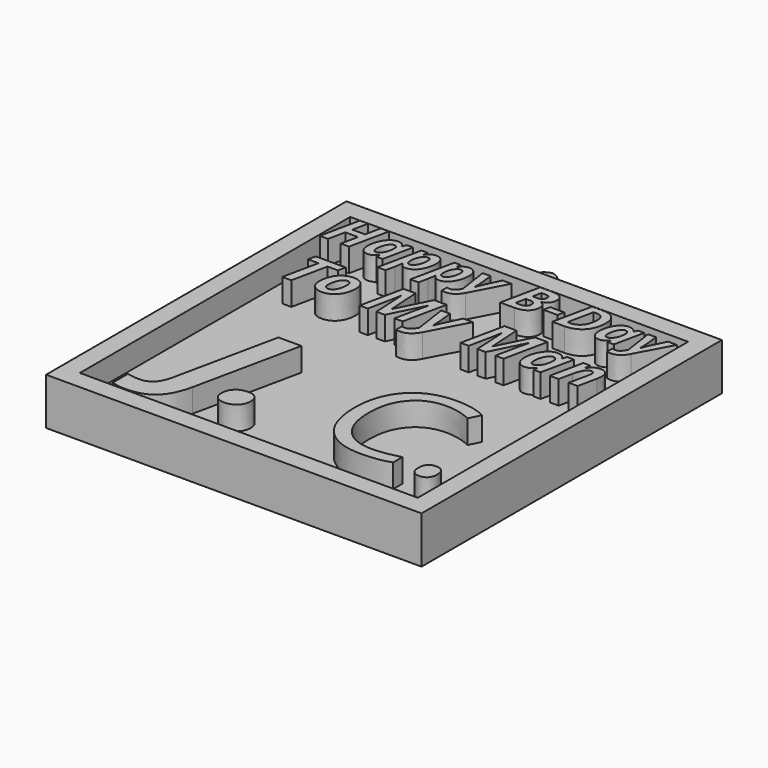
from build123d import *

# Parameters (mm, degrees)
F0_W           = 50.8
F0_H           = 50.8
F1_DEPTH       = 6.35
F2_W           = 45.72
F2_H           = 45.72
F3_DEPTH       = 3.175
F4_TEXT_SIZE   = 7.480328246
F4_TEXT_SIZE_2 = 8.230790263
F4_TEXT_SIZE_3 = 20.8935441656
F4_TEXT_SIZE_4 = 21.5266824752
F5_DEPTH       = 3.175
F6_W           = 3.175
F6_H           = 3.175
F7_DEPTH       = 3.175
F8_T1_DEPTH    = 12.7
F9_R           = 0.9525
F10_DEPTH      = 3.175


# Not quite as in the source:
# - a fillet or chamfer that OpenCascade refuses, or shapes differently, is made with other operations: its cross-section is extruded or revolved along the edge and cut away or added
# - Text() gives the source's letters only with a copy of the font that has no kerning and outlines rounded to 1/6400 em; it was checked with that copy


with BuildPart() as f1:
    # F0 (on Top) → F1 (new body)
    with BuildSketch(Plane.XY):
        Rectangle(F0_W, F0_H)
    extrude(amount=F1_DEPTH)

    # F2 (on face) → F3 (cut)
    with BuildSketch(Plane.XY.offset(6.35)):
        Rectangle(F2_W, F2_H)
    extrude(amount=-F3_DEPTH, mode=Mode.SUBTRACT)

    # F4 (on face) → F5 (join, through all)
    with BuildSketch(Plane.XY.offset(3.175)):
        with Locations((-22.86, 17.4741636629)):
            Text('Happy B-Day', F4_TEXT_SIZE, font='Open Sans', font_style=FontStyle.BOLDITALIC, text_align=(TextAlign.LEFT, TextAlign.BOTTOM))
        with Locations((-20.9547281265, 7.6553518884)):
            Text('To My Man', F4_TEXT_SIZE_2, font='Open Sans', font_style=FontStyle.BOLDITALIC, text_align=(TextAlign.LEFT, TextAlign.BOTTOM))
        with Locations((-15.4844066128, -18.3286201209)):
            Text('J.', F4_TEXT_SIZE_3, font='Open Sans', font_style=FontStyle.BOLDITALIC, text_align=(TextAlign.LEFT, TextAlign.BOTTOM))
        with Locations((3.4337516408, -18.5565501451)):
            Text('C.', F4_TEXT_SIZE_4, font='Open Sans', text_align=(TextAlign.LEFT, TextAlign.BOTTOM))
    extrude(amount=F5_DEPTH)

    # F6 (on face) → F7 (join)
    with BuildSketch(Plane(origin=(0, 25.4, 0), x_dir=(-1, 0, 0), z_dir=(0, 1, 0))):
        with Locations((0, 3.175)):
            Rectangle(F6_W, F6_H)
    extrude(amount=F7_DEPTH)

    # F8: fillet of radius 1.905 on 2 edges, made by hand

    # F8_s2 → F8_t1 (cut)
    with BuildSketch(Plane.XY.offset(-3.175)):
        with BuildLine():
            ThreePointArc((1.5875, 26.67), (1.0295384182, 28.0170384182), (-0.3175, 28.575))
            Line((-0.3175, 28.575), (1.5875, 28.575))
            Line((1.5875, 28.575), (1.5875, 26.67))
        make_face()
        with BuildLine():
            ThreePointArc((-1.5875, 26.67), (-1.0295384182, 28.0170384182), (0.3175, 28.575))
            Line((0.3175, 28.575), (-1.5875, 28.575))
            Line((-1.5875, 28.575), (-1.5875, 26.67))
        make_face()
    extrude(amount=F8_T1_DEPTH, mode=Mode.SUBTRACT)

    # F9 (on face) → F10 (cut, through all)
    with BuildSketch(Plane.XY.offset(4.7625)):
        with Locations((0, 26.67)):
            Circle(F9_R)
    extrude(amount=-F10_DEPTH, mode=Mode.SUBTRACT)


solid = f1.part
